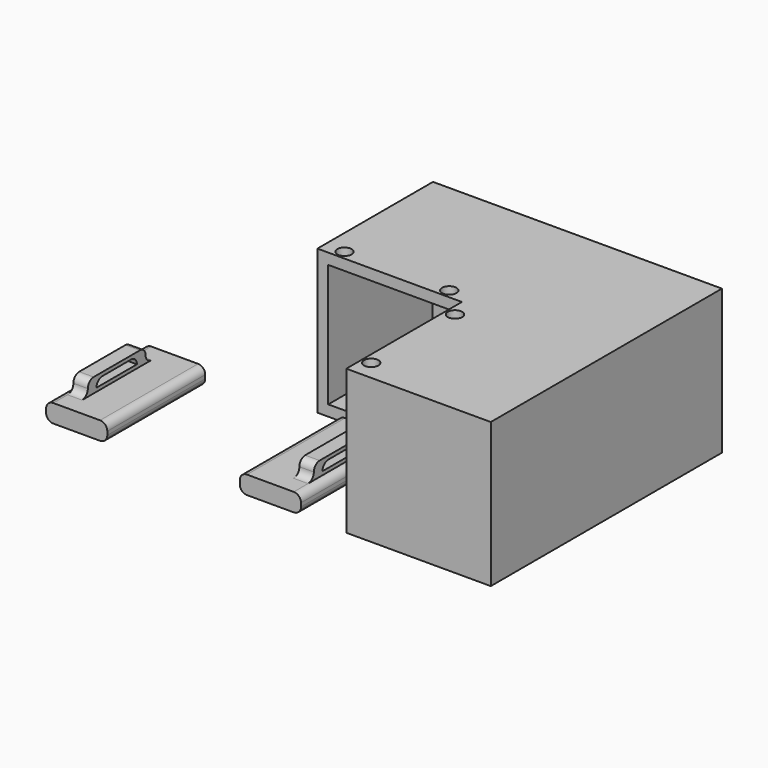
from build123d import *

# Parameters (mm, degrees)
F0_W      = 50.8
F0_H      = 50.8
F1_DEPTH  = 50.8
F4_DEPTH  = 45.72
F6_DEPTH  = 25.4
F2_W      = 43.18
F2_H      = 43.18
F7_DEPTH  = 45.72
F8_R      = 2.54
F9_DEPTH  = 25.4
F10_W     = 21.5265
F10_H     = 43.053
F11_DEPTH = 6.35
F13_DEPTH = 25.4
F15_DEPTH = 5.08
F17_DEPTH = 25.4
F18_R     = 2.53999
F19_W     = 5.3519308567
F19_H     = 34.44376681
F20_DEPTH = 25.4
F22_DEPTH = 25.4
F23_R     = 2.54
F23_2_R   = 2.54
F24_R     = 2.53999
F24_2_R   = 2.53999


# Not quite as in the source:
# - a fillet or chamfer is up to 0.001 mm smaller than in the source, because OpenCascade refuses the exact size


with BuildPart() as f1:
    # F0 (on Top) → F1 (new body)
    with BuildSketch(Plane.XY):
        with Locations((25.4, 25.4)):
            Rectangle(F0_W, F0_H)
        with Locations((-25.4, 25.4)):
            Rectangle(F0_W, F0_H)
        with Locations((25.4, -25.4)):
            Rectangle(F0_W, F0_H)
    extrude(amount=F1_DEPTH)

    # F3 (on face) → F4 (cut)
    with BuildSketch(Plane.XZ):
        Polygon((-3.81, 46.99), (-46.99, 46.99), (-3.81, 3.81), align=None)
        Polygon((-3.81, 3.81), (-46.99, 46.99), (-46.99, 3.81), align=None)
    extrude(amount=-F4_DEPTH, mode=Mode.SUBTRACT)

    # F5 (on face) → F6 (cut)
    with BuildSketch(Plane(origin=(0, 0, 46.99), x_dir=(1, 0, 0), z_dir=(0, 0, -1))):
        with BuildLine():
            ThreePointArc((-41.275, -3.175), (-42.0189487758, -1.3789487758), (-43.815, -0.635))
            ThreePointArc((-43.815, -0.635), (-45.6110512242, -4.9710512242), (-41.275, -3.175))
        make_face()
        with BuildLine():
            ThreePointArc((-4.445, -3.175), (-5.1889487758, -1.3789487758), (-6.985, -0.635))
            ThreePointArc((-6.985, -0.635), (-8.7810512242, -4.9710512242), (-4.445, -3.175))
        make_face()
    extrude(amount=-F6_DEPTH, mode=Mode.SUBTRACT)

    # F2 (on face) → F7 (cut)
    with BuildSketch(Plane(origin=(0, 0, 0), x_dir=(0, -1, 0), z_dir=(-1, 0, 0))):
        with Locations((25.4, 25.4)):
            Rectangle(F2_W, F2_H)
    extrude(amount=-F7_DEPTH, mode=Mode.SUBTRACT)

    # F8 (on face) → F9 (cut)
    with BuildSketch(Plane(origin=(0, 0, 46.99), x_dir=(1, 0, 0), z_dir=(0, 0, -1))):
        with BuildLine():
            ThreePointArc((0.635, 6.985), (3.175, 4.445), (5.715, 6.985))
            ThreePointArc((5.715, 6.985), (3.175, 9.525), (0.635, 6.985))
        make_face()
        with Locations((3.175, 43.815)):
            Circle(F8_R)
    extrude(amount=-F9_DEPTH, mode=Mode.SUBTRACT)


with BuildPart() as f11:
    # F10 (on Top) → F11 (new body)
    with BuildSketch(Plane.XY):
        with Locations((-27.0625350275, -28.8227358833)):
            Rectangle(F10_W, F10_H)
    extrude(amount=F11_DEPTH)

    # F12 (on face) → F13 (cut)
    with BuildSketch(Plane(origin=(0, -7.2962358833, 0), x_dir=(-1, 0, 0), z_dir=(0, 1, 0))):
        with BuildLine():
            ThreePointArc((34.6507850275, 0.635), (36.4468362517, 1.3789487758), (37.1907850275, 3.175))
            ThreePointArc((37.1907850275, 3.175), (32.8547338033, 4.9710512242), (34.6507850275, 0.635))
        make_face()
    extrude(amount=-F13_DEPTH, mode=Mode.SUBTRACT)

    # F14 (on face) → F15 (join)
    with BuildSketch(Plane.XY.offset(6.35)):
        Polygon((-18.8392850275, -28.8227358833), (-18.8392850275, -16.1227358833), (-23.9192850275, -16.1227358833), (-23.9192850275, -41.5227358833), (-18.8392850275, -41.5227358833), align=None)
    extrude(amount=F15_DEPTH)

    # F16 (on face) → F17 (cut)
    with BuildSketch(Plane(origin=(-23.9192850275, 0, 0), x_dir=(0, -1, 0), z_dir=(-1, 0, 0))):
        Polygon((37.7127358833, 10.16), (22.4727358833, 10.16), (35.1727358833, 7.62), (37.7127358833, 7.62), align=None)
        Polygon((35.1727358833, 7.62), (22.4727358833, 10.16), (19.9327358833, 10.16), (19.9327358833, 7.62), align=None)
    extrude(amount=-F17_DEPTH, mode=Mode.SUBTRACT)

    # F18 (radius 2.54 in the source; OpenCascade refuses exactly that, so slightly less here)
    f18_edges = [f11.edges().sort_by_distance(p)[0] for p in [
        (-21.379285, -41.522736, 6.35),
        (-21.379285, -41.522736, 11.43),
        (-21.379285, -16.122736, 11.43),
        (-21.379285, -16.122736, 6.35),
        (-21.379285, -19.932736, 10.16),
        (-21.379285, -37.712736, 10.16),
    ]]
    fillet(f18_edges, radius=F18_R)


with BuildPart() as f20:
    # F19 (on Top) → F20 (new body)
    with BuildSketch(Plane.XY):
        with Locations((-63.7897327542, -23.4408969991)):
            Rectangle(F19_W, F19_H)
    extrude(amount=F20_DEPTH)

    # F22 (cut): a face of the model
    f22_faces = [f20.faces().sort_by_distance(p)[0] for p in [
        (-63.7897327542, -23.4408969991, 25.4),
    ]]
    extrude(f22_faces, amount=-F22_DEPTH, mode=Mode.SUBTRACT)


with BuildPart() as f21_1:
    # F21: instance of F11
    add(f11.part.mirror(Plane(origin=(-61.1137673259, -23.4408969991, 12.7), x_dir=(0, 1, 0), z_dir=(1, 0, 0))))

    # F23
    f23_edges = [f21_1.edges().sort_by_distance(p)[0] for p in [
        (-84.40175, -28.822736, 6.35),
        (-84.40175, -28.822736, 0),
    ]]
    fillet(f23_edges, radius=F23_R)

    # F24#2 (radius 2.54 in the source; OpenCascade refuses exactly that, so slightly less here)
    f24_2_edges = [f21_1.edges().sort_by_distance(p)[0] for p in [
        (-105.92825, -28.822736, 6.35),
        (-105.92825, -28.822736, 0),
    ]]
    fillet(f24_2_edges, radius=F24_2_R)


with BuildPart() as f11_1:
    add(f11.part)

    # F23#2
    f23_2_edges = [f11_1.edges().sort_by_distance(p)[0] for p in [
        (-37.825785, -28.822736, 0),
        (-37.825785, -28.822736, 6.35),
    ]]
    fillet(f23_2_edges, radius=F23_2_R)

    # F24 (radius 2.54 in the source; OpenCascade refuses exactly that, so slightly less here)
    f24_edges = [f11_1.edges().sort_by_distance(p)[0] for p in [
        (-16.299285, -28.822736, 0),
        (-16.299285, -28.822736, 6.35),
    ]]
    fillet(f24_edges, radius=F24_R)


solid = Compound([f1.part, f21_1.part, f11_1.part])
